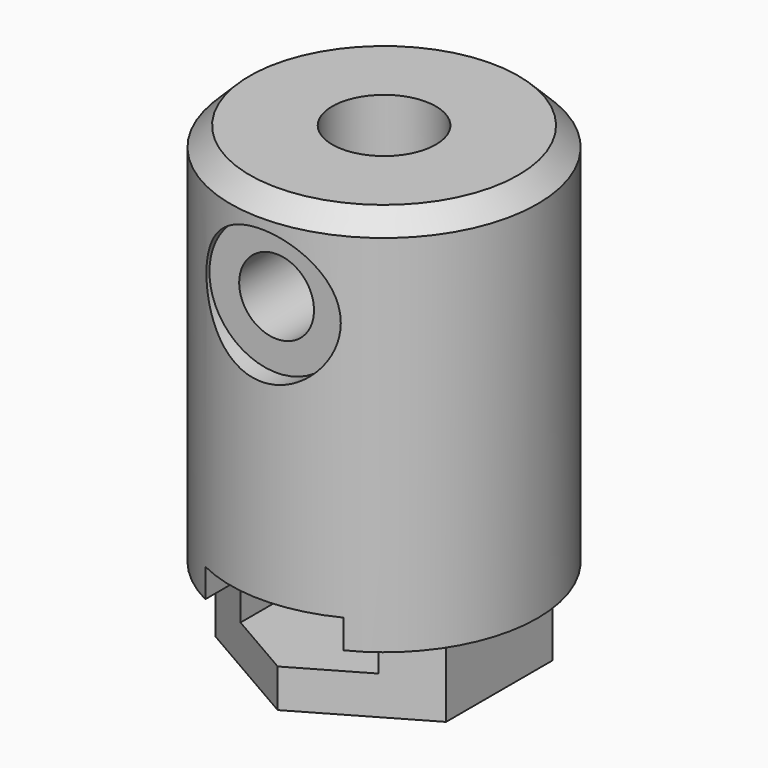
from build123d import *

# Parameters (mm, degrees)
F1_R            = 8
F2_DEPTH        = 20
F4_DEPTH        = 4
F5_R            = 2
F6_DEPTH        = 9
F9_DEPTH        = 3.5
F10_W           = 7.2
F10_H           = 3.5
F11_DEPTH       = 9
F12_SIZE        = 1
F13_R           = 2.7
F14_DEPTH       = 13
F17_D           = 3.9
F17_DEPTH       = 9
F17_CBORE_D     = 7
F17_CBORE_DEPTH = 1
F17_TIP         = 1.1716782071


with BuildPart() as f2:
    # F1 (on Top) → F2 (new body)
    with BuildSketch(Plane.XY):
        Circle(F1_R)
    extrude(amount=F2_DEPTH)

    # F3 (on face) → F4 (join)
    with BuildSketch(Plane(origin=(0, 0, 0), x_dir=(1, 0, 0), z_dir=(0, 0, -1))):
        Polygon((-6, 3.4641016151), (-6, -3.4641016151), (0, -6.9282032303), (6, -3.4641016151), (6, 3.4641016151), (0, 6.9282032303), align=None)
    extrude(amount=F4_DEPTH)

    # F5 (on face) → F6 (cut)
    with BuildSketch(Plane(origin=(0, 0, -4), x_dir=(1, 0, 0), z_dir=(0, 0, -1))):
        Circle(F5_R)
    extrude(amount=-F6_DEPTH, mode=Mode.SUBTRACT)

    # F8 (on offset) → F9 (cut)
    with BuildSketch(Plane(origin=(0, 0, -2), x_dir=(1, 0, 0), z_dir=(0, 0, -1))):
        Polygon((3.6, -2.0784609691), (3.6, 2.0784609691), (0, 4.1569219382), (-3.6, 2.0784609691), (-3.6, -2.0784609691), (0, -4.1569219382), align=None)
    extrude(amount=-F9_DEPTH, mode=Mode.SUBTRACT)

    # F10 (on Front) → F11 (cut)
    with BuildSketch(Plane.XZ):
        with Locations((0, -0.25)):
            Rectangle(F10_W, F10_H)
    extrude(amount=F11_DEPTH, mode=Mode.SUBTRACT)

    # F12
    f12_edges = [f2.edges().sort_by_distance(p)[0] for p in [
        (-8, 0, 20),
    ]]
    chamfer(f12_edges, length=F12_SIZE)

    # F13 (on face) → F14 (cut)
    with BuildSketch(Plane.XY.offset(20)):
        Circle(F13_R)
    extrude(amount=-F14_DEPTH, mode=Mode.SUBTRACT)

    # F17
    with Locations(Plane.XZ.offset(8)):
        with Locations((0, 15)):
            CounterBoreHole(F17_D / 2, F17_CBORE_D / 2, F17_CBORE_DEPTH, depth=F17_DEPTH)
            with Locations((0, 0, -(F17_DEPTH + F17_TIP / 2))):  # 118° drill point
                Cone(0, F17_D / 2, F17_TIP, mode=Mode.SUBTRACT)


solid = f2.part
